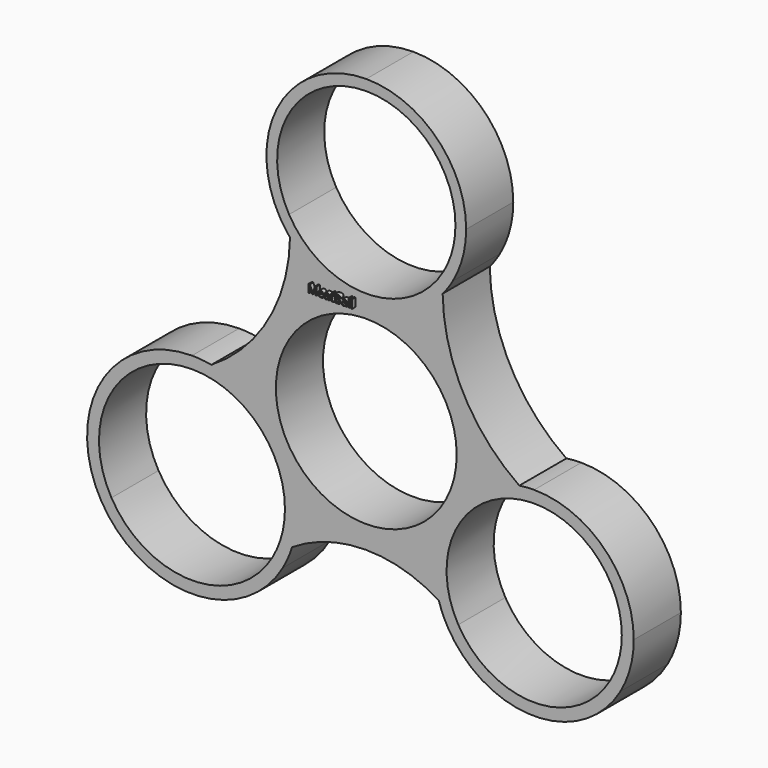
from build123d import *

# Parameters (mm, degrees)
F0_R         = 10.7476083529
F1_DEPTH     = 7
F2_TEXT_SIZE = 1.3260739959
F3_DEPTH     = 0.5


# Not quite as in the source:
# - Text() gives the source's letters only with a copy of the font that has no kerning and outlines rounded to 1/6400 em; it was checked with that copy


with BuildPart() as f1:
    # F0 (on Front) → F1 (new body)
    with BuildSketch(Plane.XZ):
        with BuildLine():
            Line((-10.2800096113, 18.0296429374), (-9.1769648825, 18.6664861086))
            ThreePointArc((-9.1769648825, 18.6664861086), (-9.1769648825, 29.263132399), (0, 34.5614555443))
            Line((0, 34.5614555443), (0, 35.8351418866))
            ThreePointArc((0, 35.8351418866), (-10.2800096113, 29.8999755702), (-10.2800096113, 18.0296429374))
        make_face()
        with BuildLine():
            ThreePointArc((-9.0648863571, 16.3010874331), (-9.0849224884, 17.4854926896), (-9.1769648825, 18.6664861086))
            Line((-9.1769648825, 18.6664861086), (-10.2800096113, 18.0296429374))
            ThreePointArc((-10.2800096113, 18.0296429374), (-9.7109848131, 17.1382749375), (-9.0648863571, 16.3010874331))
        make_face()
        with BuildLine():
            ThreePointArc((9.1769648825, 18.6664861086), (0, 13.3681629633), (-9.1769648825, 18.6664861086))
            ThreePointArc((-9.1769648825, 18.6664861086), (-9.0849224884, 17.4854926896), (-9.0648863571, 16.3010874331))
            ThreePointArc((-9.0648863571, 16.3010874331), (0.0100056117, 12.094480838), (9.0777931135, 16.3163800686))
            ThreePointArc((9.0777931135, 16.3163800686), (9.0947370255, 17.4928105422), (9.1769648825, 18.6664861086))
        make_face()
        with BuildLine():
            ThreePointArc((10.5966462905, 23.9648092538), (10.235574324, 21.2221953796), (9.1769648825, 18.6664861086))
            Line((9.1769648825, 18.6664861086), (10.2800096113, 18.0296429374))
            ThreePointArc((10.2800096113, 18.0296429374), (11.4658608566, 20.8925410968), (11.8703326328, 23.9648092538))
            ThreePointArc((11.8703326328, 23.9648092538), (8.3935926996, 32.3584019534), (0, 35.8351418866))
            Line((0, 35.8351418866), (0, 34.5614555443))
            ThreePointArc((0, 34.5614555443), (7.4929604498, 31.4577697036), (10.5966462905, 23.9648092538))
        make_face()
        with BuildLine():
            Line((10.2800096113, 18.0296429374), (9.1769648825, 18.6664861086))
            ThreePointArc((9.1769648825, 18.6664861086), (9.0947370255, 17.4928105422), (9.0777931135, 16.3163800686))
            ThreePointArc((9.0777931135, 16.3163800686), (9.7167355114, 17.1464628403), (10.2800096113, 18.0296429374))
        make_face()
        with BuildLine():
            ThreePointArc((9.0777931135, 16.3163800686), (0.0100056117, 12.094480838), (-9.0648863571, 16.3010874331))
            ThreePointArc((-9.0648863571, 16.3010874331), (-11.6257917972, 6.9101322918), (-18.4133587106, -0.0667732211))
            ThreePointArc((-18.4133587106, -0.0667732211), (-11.1241582423, -4.3592663676), (-8.2537617802, -12.3165752739))
            ThreePointArc((-8.2537617802, -12.3165752739), (-8.395614939, -14.1917353709), (-8.8179457572, -16.0242157632))
            ThreePointArc((-8.8179457572, -16.0242157632), (-0.1035543451, -13.4458661762), (8.6314199838, -15.9535997647))
            ThreePointArc((8.6314199838, -15.9535997647), (9.9425111167, -6.1949787303), (18.1824347062, -0.8048670719))
            ThreePointArc((18.1824347062, -0.8048670719), (11.556166984, 6.6528845354), (9.0777931135, 16.3163800686))
        make_face()
        Circle(F0_R, mode=Mode.SUBTRACT)
        with BuildLine():
            ThreePointArc((-8.2537617802, -12.3165752739), (-11.1241582423, -4.3592663676), (-18.4133587106, -0.0667732211))
            ThreePointArc((-18.4133587106, -0.0667732211), (-19.54593881, -0.7048303821), (-20.7185801119, -1.2658713785))
            ThreePointArc((-20.7185801119, -1.2658713785), (-12.9045524505, -4.5025476126), (-9.6678762165, -12.3165752739))
            ThreePointArc((-9.6678762165, -12.3165752739), (-10.0444198206, -15.1767079038), (-11.1483898088, -17.8419272216))
            ThreePointArc((-11.1483898088, -17.8419272216), (-10.0246094248, -16.8799401622), (-8.8179457572, -16.0242157632))
            ThreePointArc((-8.8179457572, -16.0242157632), (-8.395614939, -14.1917353709), (-8.2537617802, -12.3165752739))
        make_face()
        with BuildLine():
            ThreePointArc((-20.7185801119, -1.2658713785), (-19.54593881, -0.7048303821), (-18.4133587106, -0.0667732211))
            ThreePointArc((-18.4133587106, -0.0667732211), (-19.5609664339, 0.0943725793), (-20.7185801119, 0.1482430578))
            Line((-20.7185801119, 0.1482430578), (-20.7185801119, -1.2658713785))
        make_face()
        with BuildLine():
            ThreePointArc((19.9547614902, -0.6714216084), (19.0660897396, -0.7048301236), (18.1824347062, -0.8048670719))
            ThreePointArc((18.1824347062, -0.8048670719), (19.0549774953, -1.3790594496), (19.9547614902, -1.9095465541))
            Line((19.9547614902, -1.9095465541), (19.9547614902, -0.6714216084))
        make_face()
        with BuildLine():
            ThreePointArc((19.9547614902, -1.9095465541), (19.0549774953, -1.3790594496), (18.1824347062, -0.8048670719))
            ThreePointArc((18.1824347062, -0.8048670719), (9.9425111167, -6.1949787303), (8.6314199838, -15.9535997647))
            ThreePointArc((8.6314199838, -15.9535997647), (9.8229010209, -16.7826317108), (10.9355881414, -17.7147520901))
            ThreePointArc((10.9355881414, -17.7147520901), (10.9355881414, -7.3003077685), (19.9547614902, -2.0930856076))
            Line((19.9547614902, -2.0930856076), (19.9547614902, -1.9095465541))
        make_face()
        with BuildLine():
            ThreePointArc((-30.288770415, -17.8419272216), (-30.288770415, -6.7912233262), (-20.7185801119, -1.2658713785))
            Line((-20.7185801119, -1.2658713785), (-20.7185801119, 0.1482430578))
            ThreePointArc((-20.7185801119, 0.1482430578), (-31.5134294406, -6.084166108), (-31.5134294406, -18.5489844397))
            Line((-31.5134294406, -18.5489844397), (-30.288770415, -17.8419272216))
        make_face()
        with BuildLine():
            Line((19.9547614902, -0.6714216084), (19.9547614902, -1.9095465541))
            Line((19.9547614902, -1.9095465541), (19.9547614902, -2.0930856076))
            ThreePointArc((19.9547614902, -2.0930856076), (27.3188856924, -5.1434057271), (30.3692058119, -12.5075299293))
            ThreePointArc((30.3692058119, -12.5075299293), (30.014342227, -15.2029864639), (28.9739348391, -17.7147520901))
            Line((28.9739348391, -17.7147520901), (30.205131978, -18.4255840897))
            ThreePointArc((30.205131978, -18.4255840897), (31.3875642001, -15.5709401826), (31.7908698111, -12.5075299293))
            ThreePointArc((31.7908698111, -12.5075299293), (28.3241539467, -4.1381374728), (19.9547614902, -0.6714216084))
        make_face()
        with BuildLine():
            ThreePointArc((10.9355881414, -17.7147520901), (9.8229010209, -16.7826317108), (8.6314199838, -15.9535997647))
            ThreePointArc((8.6314199838, -15.9535997647), (9.0973244571, -17.2202278036), (9.7043910024, -18.4255840897))
            Line((9.7043910024, -18.4255840897), (10.9355881414, -17.7147520901))
        make_face()
        with BuildLine():
            ThreePointArc((-11.1483898088, -17.8419272216), (-20.7185801119, -23.3672791693), (-30.288770415, -17.8419272216))
            Line((-30.288770415, -17.8419272216), (-31.5134294406, -18.5489844397))
            ThreePointArc((-31.5134294406, -18.5489844397), (-20.7185801119, -24.7813936055), (-9.9237307831, -18.5489844397))
            Line((-9.9237307831, -18.5489844397), (-11.1483898088, -17.8419272216))
        make_face()
        with BuildLine():
            ThreePointArc((-9.9237307831, -18.5489844397), (-9.3008369407, -17.3172589189), (-8.8179457572, -16.0242157632))
            ThreePointArc((-8.8179457572, -16.0242157632), (-10.0246094248, -16.8799401622), (-11.1483898088, -17.8419272216))
            Line((-11.1483898088, -17.8419272216), (-9.9237307831, -18.5489844397))
        make_face()
        with BuildLine():
            ThreePointArc((28.9739348391, -17.7147520901), (19.9547614902, -22.9219742509), (10.9355881414, -17.7147520901))
            Line((10.9355881414, -17.7147520901), (9.7043910024, -18.4255840897))
            ThreePointArc((9.7043910024, -18.4255840897), (19.9547614902, -24.3436382501), (30.205131978, -18.4255840897))
            Line((30.205131978, -18.4255840897), (28.9739348391, -17.7147520901))
        make_face()
    extrude(amount=F1_DEPTH)

    # F2 (on face) → F3 (join)
    with BuildSketch(Plane.XZ.offset(7)):
        with Locations((-6.5879360773, 11.5527566522)):
            Text('MeatBall', F2_TEXT_SIZE, font='Open Sans', text_align=(TextAlign.LEFT, TextAlign.BOTTOM))
    extrude(amount=F3_DEPTH)


solid = f1.part
